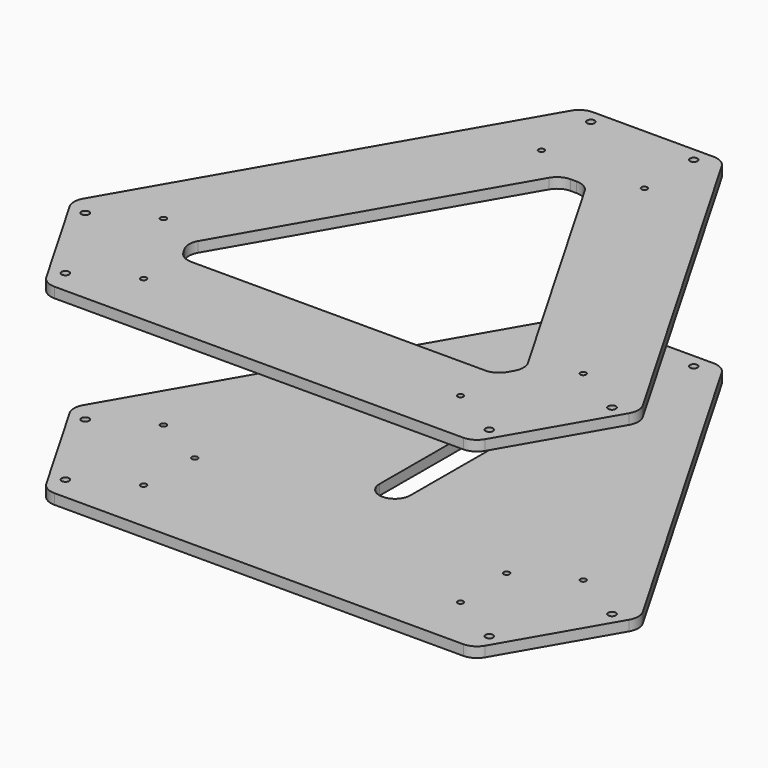
from build123d import *

# Parameters (mm, degrees)
F0_R     = 2.2
F0_R_2   = 1.7
F1_DEPTH = 6
F3_R     = 2.2
F3_R_2   = 1.7
F4_DEPTH = 6
F5_R     = 10
F5_2_R   = 10


# Not quite as in the source:
# - a feature names something its author has since deleted; it is built from what else it names


with BuildPart() as f1:
    # F0 (on Top) → F1 (new body)
    with BuildSketch(Plane.XY):
        Polygon((-41, 168.0089283342), (-166, -48.4974226119), (-125, -119.5115057223), (125, -119.5115057223), (166, -48.4974226119), (41, 168.0089283342), align=None)
        with Locations((-123.5717967697, -105.9852262806)):
            Circle(F0_R, mode=Mode.SUBTRACT)
        with Locations((-92.3948822335, -87.9852262806)):
            Circle(F0_R_2, mode=Mode.SUBTRACT)
        with Locations((-153.5717967697, -54.0237020536)):
            Circle(F0_R, mode=Mode.SUBTRACT)
        with Locations((-122.3948822335, -36.0237020536)):
            Circle(F0_R_2, mode=Mode.SUBTRACT)
        Polygon((99.027368774, -48.4974226119), (91.513684387, -61.5115057223), (-91.513684387, -61.5115057223), (-99.027368774, -48.4974226119), (-7.513684387, 110.0089283342), (7.513684387, 110.0089283342), align=None, mode=Mode.SUBTRACT)
        with Locations((123.5717967697, -105.9852262806)):
            Circle(F0_R, mode=Mode.SUBTRACT)
        with Locations((92.3948822335, -87.9852262806)):
            Circle(F0_R_2, mode=Mode.SUBTRACT)
        with Locations((153.5717967697, -54.0237020536)):
            Circle(F0_R, mode=Mode.SUBTRACT)
        with Locations((122.3948822335, -36.0237020536)):
            Circle(F0_R_2, mode=Mode.SUBTRACT)
        with Locations((-30, 124.0089283342)):
            Circle(F0_R_2, mode=Mode.SUBTRACT)
        with Locations((-30, 160.0089283342)):
            Circle(F0_R, mode=Mode.SUBTRACT)
        with Locations((30, 124.0089283342)):
            Circle(F0_R_2, mode=Mode.SUBTRACT)
        with Locations((30, 160.0089283342)):
            Circle(F0_R, mode=Mode.SUBTRACT)
    extrude(amount=F1_DEPTH)

    # F5
    f5_edges = [f1.edges().sort_by_distance(p)[0] for p in [
        (-125, -119.511506, 3),
        (-166, -48.497423, 3),
        (125, -119.511506, 3),
        (166, -48.497423, 3),
        (-41, 168.008928, 3),
        (41, 168.008928, 3),
        (-99.027369, -48.497423, 3),
        (-91.513684, -61.511506, 3),
        (-7.513684, 110.008928, 3),
        (7.513684, 110.008928, 3),
        (99.027369, -48.497423, 3),
        (91.513684, -61.511506, 3),
    ]]
    fillet(f5_edges, radius=F5_R)


with BuildPart() as f4:
    # F3 (on offset) → F4 (new body)
    with BuildSketch(Plane(origin=(0, 0, -100), x_dir=(1, 0, 0), z_dir=(0, 0, -1))):
        Polygon((125, 119.5115057223), (-125, 119.5115057223), (-166, 48.4974226119), (-41, -168.0089283342), (41, -168.0089283342), (166, 48.4974226119), align=None)
        with Locations((-30, -160.0089283342)):
            Circle(F3_R, mode=Mode.SUBTRACT)
        with Locations((-30, -124.0089283342)):
            Circle(F3_R_2, mode=Mode.SUBTRACT)
        with BuildLine():
            Line((8.7580333745, 20.0241934108), (8.9999674821, -69.9754814103))
            ThreePointArc((8.9999674821, -69.9754814103), (0.0241934108, -78.9996423031), (-8.9999674821, -70.0238682318))
            Line((-8.9999674821, -70.0238682318), (-9.2419015897, 19.9758065892))
            ThreePointArc((-9.2419015897, 19.9758065892), (-0.2661275183, 28.9999674821), (8.7580333745, 20.0241934108))
        make_face(mode=Mode.SUBTRACT)
        with Locations((30, -160.0089283342)):
            Circle(F3_R, mode=Mode.SUBTRACT)
        with Locations((30, -124.0089283342)):
            Circle(F3_R_2, mode=Mode.SUBTRACT)
        with Locations((0, -105)):
            Circle(F3_R_2, mode=Mode.SUBTRACT)
        with Locations((-122.3948822335, 36.0237020536)):
            Circle(F3_R_2, mode=Mode.SUBTRACT)
        with Locations((-153.5717967697, 54.0237020536)):
            Circle(F3_R, mode=Mode.SUBTRACT)
        with Locations((-90.9326673974, 52.5)):
            Circle(F3_R_2, mode=Mode.SUBTRACT)
        with Locations((-92.3948822335, 87.9852262806)):
            Circle(F3_R_2, mode=Mode.SUBTRACT)
        with Locations((-123.5717967697, 105.9852262806)):
            Circle(F3_R, mode=Mode.SUBTRACT)
        with Locations((122.3948822335, 36.0237020536)):
            Circle(F3_R_2, mode=Mode.SUBTRACT)
        with Locations((90.9326673974, 52.5)):
            Circle(F3_R_2, mode=Mode.SUBTRACT)
        with Locations((153.5717967697, 54.0237020536)):
            Circle(F3_R, mode=Mode.SUBTRACT)
        with Locations((92.3948822335, 87.9852262806)):
            Circle(F3_R_2, mode=Mode.SUBTRACT)
        with Locations((123.5717967697, 105.9852262806)):
            Circle(F3_R, mode=Mode.SUBTRACT)
    extrude(amount=F4_DEPTH)

    # F5#2
    f5_2_edges = [f4.edges().sort_by_distance(p)[0] for p in [
        (125, -119.511506, -103),
        (166, -48.497423, -103),
        (-125, -119.511506, -103),
        (-166, -48.497423, -103),
        (-41, 168.008928, -103),
        (41, 168.008928, -103),
    ]]
    fillet(f5_2_edges, radius=F5_2_R)


solid = Compound([f1.part, f4.part])
